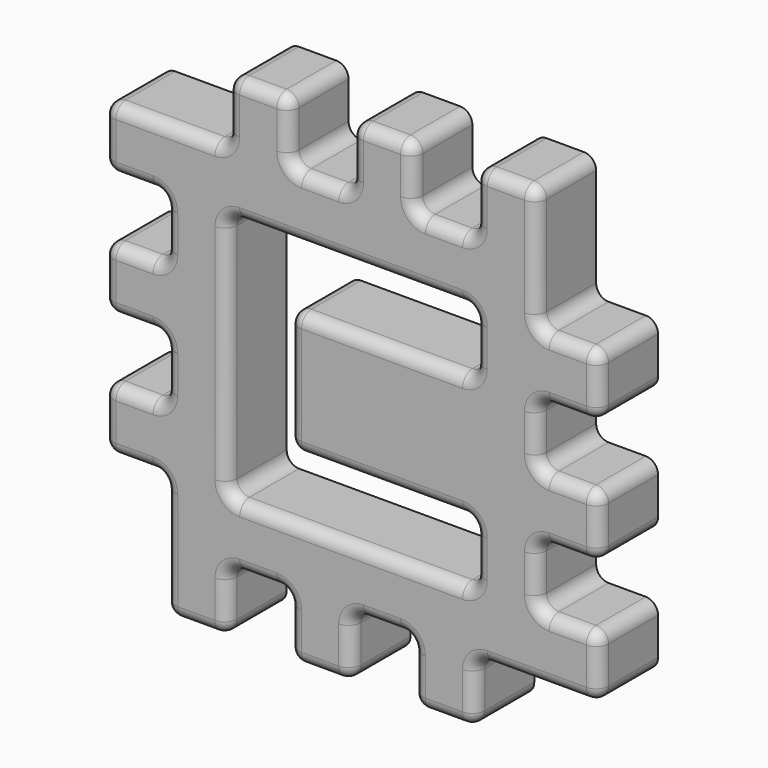
from build123d import *

# Parameters (mm, degrees)
F0_W     = 5
F0_H     = 5
F1_DEPTH = 6
F2_F1_R  = 1
F2_F2_R  = 1
F3_R     = 1


with BuildPart() as f1:
    # F0 (on Front) → F1 (new body)
    with BuildSketch(Plane.XZ):
        Polygon((-15, -10), (-15, -15), (-10, -15), (-5, -15), (0, -15), (5, -15), (10, -15), (15, -15), (15, -10), (15, -5), (15, 0), (15, 5), (15, 10), (15, 15), (10, 15), (5, 15), (0, 15), (-5, 15), (-10, 15), (-15, 15), (-15, 10), (-15, 5), (-15, 0), (-15, -5), align=None)
        Polygon((-5, 10), (10, 10), (10, 5), (-5, 5), (-5, -5), (10, -5), (10, -10), (-5, -10), (-10, -10), (-10, -5), (-10, 5), (-10, 10), align=None, mode=Mode.SUBTRACT)
        with Locations((-12.5, -17.5)):
            Rectangle(F0_W, F0_H)
        with Locations((-17.5, -7.5)):
            Rectangle(F0_W, F0_H)
        with Locations((-2.5, -17.5)):
            Rectangle(F0_W, F0_H)
        with Locations((-17.5, 2.5)):
            Rectangle(F0_W, F0_H)
        with Locations((7.5, -17.5)):
            Rectangle(F0_W, F0_H)
        with Locations((-17.5, 12.5)):
            Rectangle(F0_W, F0_H)
        with Locations((17.5, -12.5)):
            Rectangle(F0_W, F0_H)
        with Locations((-7.5, 17.5)):
            Rectangle(F0_W, F0_H)
        with Locations((17.5, -2.5)):
            Rectangle(F0_W, F0_H)
        with Locations((2.5, 17.5)):
            Rectangle(F0_W, F0_H)
        with Locations((17.5, 7.5)):
            Rectangle(F0_W, F0_H)
        with Locations((12.5, 17.5)):
            Rectangle(F0_W, F0_H)
    extrude(amount=F1_DEPTH)

    # F2: fillet of radius 1 on 10 edges, made by hand

    # F2_f1
    f2_f1_edges = [f1.edges().sort_by_distance(p)[0] for p in [
        (-10, -3, 10),
        (10, -3, 10),
        (10, -3, -5),
        (10, -3, 5),
        (10, -3, -10),
        (-10, -3, -10),
    ]]
    fillet(f2_f1_edges, radius=F2_F1_R)

    # F2_f2
    f2_f2_edges = [f1.edges().sort_by_distance(p)[0] for p in [
        (-5, -3, -5),
        (-5, -3, 5),
        (2, -6, -5),
        (-5, -6, 0),
        (9.7071067812, -6, -5.2928932188),
    ]]
    fillet(f2_f2_edges, radius=F2_F2_R)

    # F3
    f3_edges = [f1.edges().sort_by_distance(p)[0] for p in [
        (-5, -6, 17.5),
        (-15, -6, 15),
        (7.5, -6, 15),
        (5, -6, 17.5),
        (10, -3, 15),
        (0, -3, 15),
        (-2.5, -6, 15),
        (-10, -3, 15),
        (-7.5, -6, 20),
        (-10, -3, 20),
        (-15, -6, 7.5),
        (-5, -3, 15),
        (5, -3, 15),
        (5, -3, 20),
        (-5, -3, 20),
        (0, -3, 20),
        (10, -3, 20),
        (-20, -3, 15),
        (-20, -6, 12.5),
        (-20, -3, 10),
        (2.5, -6, -4),
        (-4, -6, 0),
        (10.414214, -6, -4.585786),
        (2.5, -6, 4),
        (11, -6, -7.5),
        (10.414214, -6, 4.585786),
        (10.414214, -6, -10.414214),
        (11, -6, 7.5),
        (0, -6, -11),
        (10.414214, -6, 10.414214),
        (-10.414214, -6, -10.414214),
        (0, -6, 11),
        (-11, -6, 0),
        (-10.414214, -6, 10.414214),
        (-12.5, -6, -20),
        (-10, -6, -17.5),
        (-7.5, -6, -15),
        (-5, -6, -17.5),
        (-2.5, -6, -20),
        (0, -6, -17.5),
        (2.5, -6, -15),
        (5, -6, -17.5),
        (7.5, -6, -20),
        (10, -6, -17.5),
        (15, -6, -15),
        (20, -6, -12.5),
        (17.5, -6, -10),
        (15, -6, -7.5),
        (17.5, -6, -5),
        (20, -6, -2.5),
        (17.5, -6, 0),
        (15, -6, 2.5),
        (17.5, -6, 5),
        (20, -6, 7.5),
        (17.5, -6, 10),
        (15, -6, 15),
        (12.5, -6, 20),
        (10, -6, 17.5),
        (2.5, -6, 20),
        (0, -6, 17.5),
        (-10, -6, 17.5),
        (-17.5, -6, 10),
        (-17.5, -6, 5),
        (-20, -6, 2.5),
        (-17.5, -6, 0),
        (-15, -6, -2.5),
        (-17.5, -6, -5),
        (-20, -6, -7.5),
        (-17.5, -6, -10),
        (-15, -6, -15),
        (-15, -3, 5),
        (-20, -3, 5),
        (-20, -3, 0),
        (-15, -3, -5),
        (-20, -3, -5),
        (-15, -3, 0),
        (-15, -3, 10),
        (-20, -3, -10),
        (-15, -3, -10),
        (-15, -3, -20),
        (-5, -3, -15),
        (5, -3, -15),
        (20, -3, -15),
        (10, -3, -20),
        (5, -3, -20),
        (0, -3, -20),
        (-5, -3, -20),
        (-10, -3, -20),
        (-10, -3, -15),
        (0, -3, -15),
        (10, -3, -15),
        (20, -3, -10),
        (15, -3, -10),
        (20, -3, 10),
        (15, -3, 20),
        (15, -3, -5),
        (20, -3, -5),
        (15, -3, 10),
        (15, -3, 5),
        (15, -3, 0),
        (20, -3, 0),
        (20, -3, 5),
    ]]
    fillet(f3_edges, radius=F3_R)


solid = f1.part
